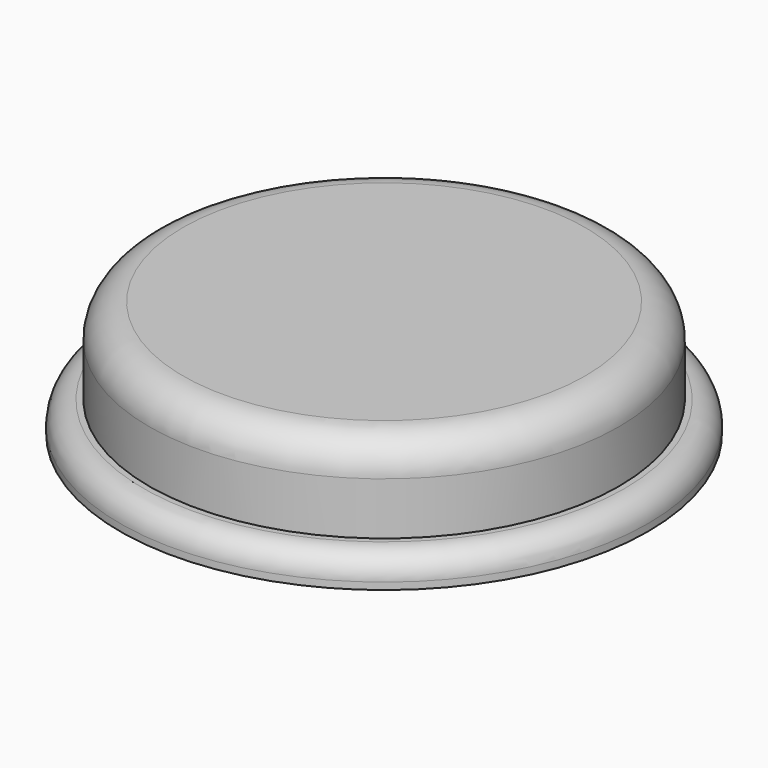
from build123d import *

# Parameters (mm, degrees)
F0_R     = 51.2202453394
F2_DEPTH = 25.4
F3_R     = 7.3585229381
F0_R_2   = 57.5702453394
F4_DEPTH = 6.604
F5_R     = 5.08


# Not quite as in the source:
# - the program builds the solid bodies; features that only make, move or delete a surface that nothing else refers to are left out


with BuildPart() as f2:
    # F0 (on Top) → F2 (new body)
    with BuildSketch(Plane.XY):
        Circle(F0_R)
    extrude(amount=F2_DEPTH)

    # F3
    f3_edges = [f2.edges().sort_by_distance(p)[0] for p in [
        (-51.220245, 0, 25.4),
    ]]
    fillet(f3_edges, radius=F3_R)

    # F0 (on Top) → F4 (join)
    with BuildSketch(Plane.XY):
        Circle(F0_R_2)
        Circle(F0_R, mode=Mode.SUBTRACT)
    extrude(amount=F4_DEPTH)

    # F5
    f5_edges = [f2.edges().sort_by_distance(p)[0] for p in [
        (-57.570245, 0, 6.604),
    ]]
    fillet(f5_edges, radius=F5_R)


solid = f2.part
